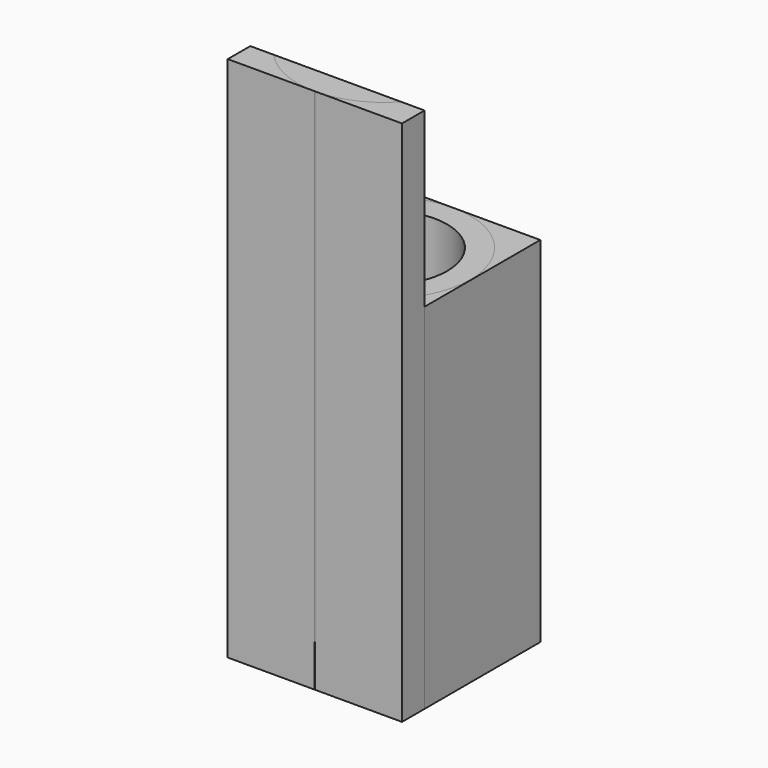
from build123d import *

# Parameters (mm, degrees)
F1_DEPTH = 84
F2_DEPTH = 125
F3_DEPTH = 115
F5_DEPTH = 74
F6_DEPTH = 115


with BuildPart() as f1:
    # F0 (on Top) → F1 (new body)
    with BuildSketch(Plane.XY):
        with BuildLine():
            ThreePointArc((20.5, 0), (19.1142782295, -7.4090733406), (15.1444519252, -13.8164965127))
            Line((15.1444519252, -13.8164965127), (20.6728133691, -13.8164965127))
            Line((20.6728133691, -13.8164965127), (20.6728133691, 20.4998192933))
            Line((20.6728133691, 20.4998192933), (0.0860752209, 20.4998192933))
            ThreePointArc((0.0860752209, 20.4998192933), (14.5260893228, 14.4652248163), (20.5, 0))
        make_face()
    extrude(amount=F1_DEPTH)


with BuildPart() as f1b:
    # F0 (on Top) → F1, piece 2 (new body)
    with BuildSketch(Plane.XY):
        with BuildLine():
            ThreePointArc((-15.1444519252, -13.8164965127), (-18.7721768027, 8.2374375924), (-0.0860752209, 20.4998192933))
            Line((-0.0860752209, 20.4998192933), (-20.6728133691, 20.4998192933))
            Line((-20.6728133691, 20.4998192933), (-20.6728133691, -13.8164965127))
            Line((-20.6728133691, -13.8164965127), (-15.1444519252, -13.8164965127))
        make_face()
    extrude(amount=F1_DEPTH)


with BuildPart() as f2:
    # F0 (on Top) → F2 (new body)
    with BuildSketch(Plane.XY):
        with BuildLine():
            Line((-20.6728133691, -20.4998192933), (-0.0860752209, -20.4998192933))
            ThreePointArc((-0.0860752209, -20.4998192933), (-8.3161854317, -18.7374240456), (-15.1444519252, -13.8164965127))
            Line((-15.1444519252, -13.8164965127), (-20.6728133691, -13.8164965127))
            Line((-20.6728133691, -13.8164965127), (-20.6728133691, -20.4998192933))
        make_face()
    extrude(amount=F2_DEPTH)


with BuildPart() as f2b:
    # F0 (on Top) → F2, piece 2 (new body)
    with BuildSketch(Plane.XY):
        with BuildLine():
            Line((20.6728133691, -13.8164965127), (15.1444519252, -13.8164965127))
            ThreePointArc((15.1444519252, -13.8164965127), (8.3161854317, -18.7374240456), (0.0860752209, -20.4998192933))
            Line((0.0860752209, -20.4998192933), (20.6728133691, -20.4998192933))
            Line((20.6728133691, -20.4998192933), (20.6728133691, -13.8164965127))
        make_face()
    extrude(amount=F2_DEPTH)


with BuildPart() as f3:
    # F0 (on Top) → F3 (new body)
    with BuildSketch(Plane.XY):
        with BuildLine():
            ThreePointArc((0.0860752209, -20.4998192933), (8.3161854317, -18.7374240456), (15.1444519252, -13.8164965127))
            Line((15.1444519252, -13.8164965127), (5.839899324, -13.8164965127))
            ThreePointArc((5.839899324, -13.8164965127), (0, -15), (-5.839899324, -13.8164965127))
            Line((-5.839899324, -13.8164965127), (-15.1444519252, -13.8164965127))
            ThreePointArc((-15.1444519252, -13.8164965127), (-8.3161854317, -18.7374240456), (-0.0860752209, -20.4998192933))
            Line((-0.0860752209, -20.4998192933), (0.0860752209, -20.4998192933))
        make_face()
    extrude(amount=F3_DEPTH)

    # F0 (on Top) → F6 (join)
    with BuildSketch(Plane.XY):
        with BuildLine():
            ThreePointArc((-5.839899324, -13.8164965127), (0, -15), (5.839899324, -13.8164965127))
            Line((5.839899324, -13.8164965127), (-5.839899324, -13.8164965127))
        make_face()
    extrude(amount=F6_DEPTH)


with BuildPart() as f2b_1:
    # F4: moved
    add(f2b.part.moved(Location((0, 0, -10))))


with BuildPart() as f2_1:
    # F4: moved
    add(f2.part.moved(Location((0, 0, -10))))


with BuildPart() as f1b_1:
    # F4: moved
    add(f1b.part.moved(Location((0, 0, -10))))


with BuildPart() as f1_1:
    # F4: moved
    add(f1.part.moved(Location((0, 0, -10))))


with BuildPart() as f5:
    # F0 (on Top) → F5 (new body)
    with BuildSketch(Plane.XY):
        with BuildLine():
            Line((5.839899324, -13.8164965127), (15.1444519252, -13.8164965127))
            ThreePointArc((15.1444519252, -13.8164965127), (19.1142782295, -7.4090733406), (20.5, 0))
            ThreePointArc((20.5, 0), (14.5260893228, 14.4652248163), (0.0860752209, 20.4998192933))
            Line((0.0860752209, 20.4998192933), (-0.0860752209, 20.4998192933))
            ThreePointArc((-0.0860752209, 20.4998192933), (-18.7721768027, 8.2374375924), (-15.1444519252, -13.8164965127))
            Line((-15.1444519252, -13.8164965127), (-5.839899324, -13.8164965127))
            ThreePointArc((-5.839899324, -13.8164965127), (-8.2885918629, 12.501969642), (15, 0))
            ThreePointArc((15, 0), (12.501969642, -8.2885918629), (5.839899324, -13.8164965127))
        make_face()
    extrude(amount=F5_DEPTH)


solid = Compound([f3.part, f2b_1.part, f2_1.part, f1b_1.part, f1_1.part, f5.part])
